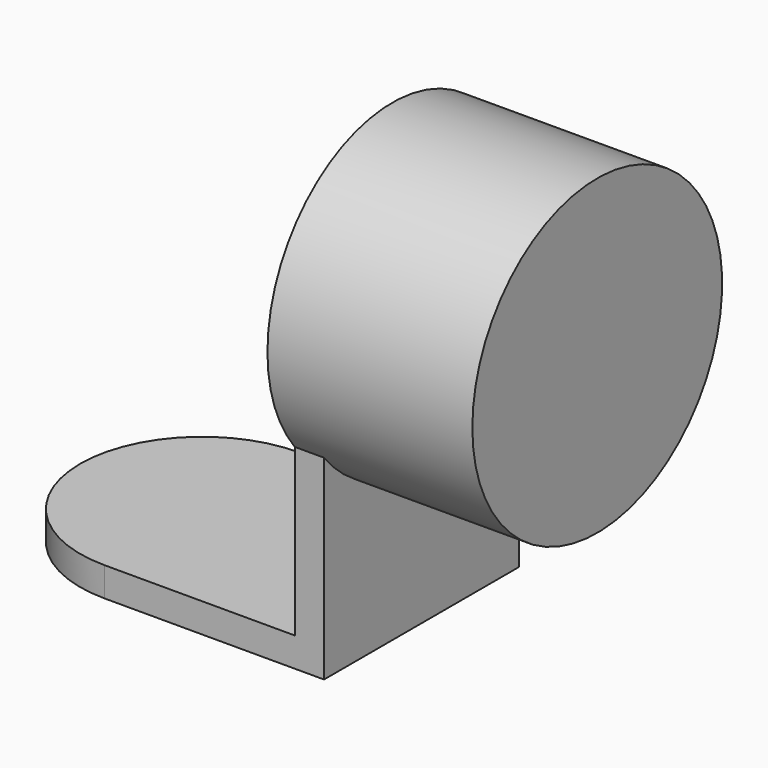
from build123d import *

# Parameters (mm, degrees)
F0_W     = 35
F0_H     = 25
F1_DEPTH = 3
F2_W     = 3
F2_H     = 25
F3_DEPTH = 40
F4_R     = 12.49999
F5_R     = 12.49999
F6_R     = 16
F7_DEPTH = 21
F8_R     = 14.5
F9_DEPTH = 18


# Not quite as in the source:
# - a fillet or chamfer is up to 0.001 mm smaller than in the source, because OpenCascade refuses the exact size


with BuildPart() as f1:
    # F0 (on Top) → F1 (new body)
    with BuildSketch(Plane.XY):
        Rectangle(F0_W, F0_H)
    extrude(amount=F1_DEPTH)

    # F2 (on Top) → F3 (join)
    with BuildSketch(Plane.XY):
        with Locations((16, 0)):
            Rectangle(F2_W, F2_H)
    extrude(amount=F3_DEPTH)

    # F4 (radius 12.5 in the source; OpenCascade refuses exactly that, so slightly less here)
    f4_edges = [f1.edges().sort_by_distance(p)[0] for p in [
        (-17.5, 12.5, 1.5),
        (-17.5, -12.5, 1.5),
    ]]
    fillet(f4_edges, radius=F4_R)

    # F5 (radius 12.5 in the source; OpenCascade refuses exactly that, so slightly less here)
    f5_edges = [f1.edges().sort_by_distance(p)[0] for p in [
        (16, 12.5, 40),
        (16, -12.5, 40),
    ]]
    fillet(f5_edges, radius=F5_R)

    # F6 (on face) → F7 (join)
    with BuildSketch(Plane(origin=(14.5, 0, 0), x_dir=(0, -1, 0), z_dir=(-1, 0, 0))):
        with Locations((0, 30)):
            Circle(F6_R)
    extrude(amount=-F7_DEPTH)

    # F8 (on face) → F9 (cut)
    with BuildSketch(Plane(origin=(14.5, 0, 0), x_dir=(0, -1, 0), z_dir=(-1, 0, 0))):
        with Locations((0, 30)):
            Circle(F8_R)
    extrude(amount=-F9_DEPTH, mode=Mode.SUBTRACT)


solid = f1.part
